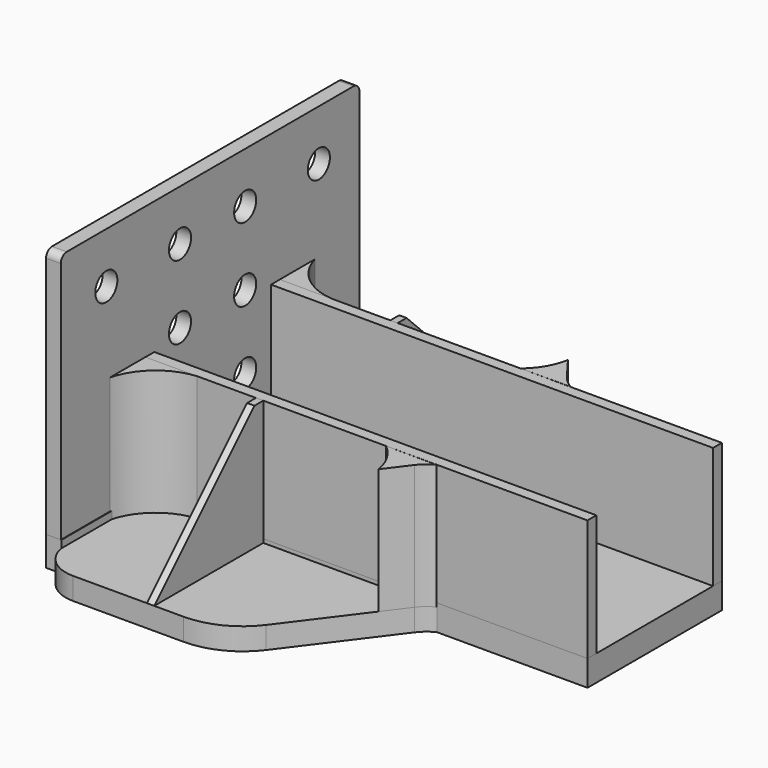
from build123d import *

# Parameters (mm, degrees)
F1_DEPTH   = 3.81
F2_W       = 2.54
F2_H       = 64.319235925
F3_DEPTH   = 44.45
F4_R       = 1.27
F5_R       = 1.27
F6_W       = 76.1874727905
F6_H       = 1.905
F7_DEPTH   = 25.4
F9_DEPTH   = 21.59
F11_DEPTH  = 21.59
F12_W      = 1.27
F12_H      = 23.495
F13_DEPTH  = 21.59
F14_SIZE   = 21.58999
F14_2_SIZE = 21.58999
F15_R      = 2.38125
F16_DEPTH  = 2.541
F17_W      = 78.74
F17_H      = 28.956
F18_DEPTH  = 4.445
F19_W      = 2.63135281
F19_H      = 18.218235925
F20_DEPTH  = 5.08


# Not quite as in the source:
# - a fillet or chamfer is up to 0.001 mm smaller than in the source, because OpenCascade refuses the exact size


with BuildPart() as f1:
    # F0 (on Top) → F1 (new body)
    with BuildSketch(Plane.XY):
        with BuildLine():
            Line((-38.1, 31.623), (-38.1, 12.573))
            Line((-38.1, 12.573), (12.7, 12.573))
            Line((12.7, 12.573), (38.1, 12.573))
            Line((38.1, 12.573), (38.1, 13.843))
            Line((38.1, 13.843), (14.9225, 13.843))
            ThreePointArc((14.9225, 13.843), (12.0826936686, 14.5133873372), (9.8425, 16.383))
            Line((9.8425, 16.383), (-2.54, 32.893))
            ThreePointArc((-2.54, 32.893), (-7.0203873372, 36.6322253257), (-12.7, 37.973))
            Line((-12.7, 37.973), (-31.75, 37.973))
            ThreePointArc((-31.75, 37.973), (-36.2401280605, 36.1131280605), (-38.1, 31.623))
        make_face()
    extrude(amount=F1_DEPTH)


with BuildPart() as f1b:
    # F0 (on Top) → F1, piece 2 (new body)
    with BuildSketch(Plane.XY):
        with BuildLine():
            Line((14.9225, -13.843), (38.1, -13.843))
            Line((38.1, -13.843), (38.1, -12.573))
            Line((38.1, -12.573), (12.7, -12.573))
            Line((12.7, -12.573), (-38.1, -12.573))
            Line((-38.1, -12.573), (-38.1, -31.623))
            ThreePointArc((-38.1, -31.623), (-36.2401280605, -36.1131280605), (-31.75, -37.973))
            Line((-31.75, -37.973), (-12.7, -37.973))
            ThreePointArc((-12.7, -37.973), (-7.0203873372, -36.6322253257), (-2.54, -32.893))
            Line((-2.54, -32.893), (9.8425, -16.383))
            ThreePointArc((9.8425, -16.383), (12.0826936686, -14.5133873372), (14.9225, -13.843))
        make_face()
    extrude(amount=F1_DEPTH)


with BuildPart() as f3:
    # F2 (on face) → F3 (new body)
    with BuildSketch(Plane.XY.offset(3.81)):
        with Locations((-39.37, -0.5366179625)):
            Rectangle(F2_W, F2_H)
    extrude(amount=F3_DEPTH)

    # F4
    f4_edges = [f3.edges().sort_by_distance(p)[0] for p in [
        (-39.37, 31.623, 48.26),
    ]]
    fillet(f4_edges, radius=F4_R)

    # F5
    f5_edges = [f3.edges().sort_by_distance(p)[0] for p in [
        (-39.37, -32.696236, 48.26),
    ]]
    fillet(f5_edges, radius=F5_R)

    # F15 (on face) → F16 (cut, through all)
    with BuildSketch(Plane.YZ.offset(-38.1)):
        with Locations((22.89175, 39.52875)):
            Circle(F15_R)
        with Locations((7.01675, 39.52875)):
            Circle(F15_R)
        with Locations((7.01675, 26.82875)):
            Circle(F15_R)
        with Locations((7.01675, 14.12875)):
            Circle(F15_R)
        with Locations((-22.89175, 39.52875)):
            Circle(F15_R)
        with Locations((-7.01675, 26.82875)):
            Circle(F15_R)
        with Locations((-7.01675, 14.12875)):
            Circle(F15_R)
        with Locations((-7.01675, 39.52875)):
            Circle(F15_R)
    extrude(amount=-F16_DEPTH, mode=Mode.SUBTRACT)


with BuildPart() as f7:
    # F6 (on Top) → F7 (new body)
    with BuildSketch(Plane.XY):
        with Locations((0.0062636048, 13.5255)):
            Rectangle(F6_W, F6_H)
    extrude(amount=F7_DEPTH)


with BuildPart() as f7b:
    # F6 (on Top) → F7, piece 2 (new body)
    with BuildSketch(Plane.XY):
        with Locations((0.0062636048, -13.5255)):
            Rectangle(F6_W, F6_H)
    extrude(amount=F7_DEPTH)


with BuildPart() as f9:
    # F8 (on face) → F9 (new body)
    with BuildSketch(Plane.XY.offset(3.81)):
        with BuildLine():
            ThreePointArc((-29.2110200971, 14.478), (-34.8634746859, 16.8788696345), (-38.1, 22.098))
            Line((-38.1, 22.098), (-38.1, 14.4734261557))
            Line((-38.1, 14.4734261557), (-29.2110200971, 14.478))
        make_face()
    extrude(amount=F9_DEPTH)


with BuildPart() as f9b:
    # F8 (on face) → F9, piece 2 (new body)
    with BuildSketch(Plane.XY.offset(3.81)):
        with BuildLine():
            Line((-38.1, -14.4734261557), (-38.1, -22.098))
            ThreePointArc((-38.1, -22.098), (-34.8634746859, -16.8788696345), (-29.2110200971, -14.478))
            Line((-29.2110200971, -14.478), (-38.1, -14.4734261557))
        make_face()
    extrude(amount=F9_DEPTH)


with BuildPart() as f11:
    # F10 (on face) → F11 (new body)
    with BuildSketch(Plane.XY.offset(3.81)):
        with BuildLine():
            ThreePointArc((6.8367980262, 20.3906026317), (5.6419248641, 17.1304778187), (3.4012782853, 14.478))
            Line((3.4012782853, 14.478), (12.0826936686, 14.5133873372))
            ThreePointArc((12.0826936686, 14.5133873372), (10.8537537608, 15.3177765137), (9.8425, 16.383))
            Line((9.8425, 16.383), (6.8367980262, 20.3906026317))
        make_face()
    extrude(amount=F11_DEPTH)


with BuildPart() as f11b:
    # F10 (on face) → F11, piece 2 (new body)
    with BuildSketch(Plane.XY.offset(3.81)):
        with BuildLine():
            Line((12.0826936686, -14.5133873372), (3.4012782853, -14.478))
            ThreePointArc((3.4012782853, -14.478), (5.6419248641, -17.1304778187), (6.8367980262, -20.3906026317))
            Line((6.8367980262, -20.3906026317), (9.8425, -16.383))
            ThreePointArc((9.8425, -16.383), (10.8537537608, -15.3177765137), (12.0826936686, -14.5133873372))
        make_face()
    extrude(amount=F11_DEPTH)


with BuildPart() as f13:
    # F12 (on face) → F13 (new body)
    with BuildSketch(Plane.XY.offset(3.81)):
        with Locations((-18.415, 26.2255)):
            Rectangle(F12_W, F12_H)
    extrude(amount=F13_DEPTH)

    # F14 (size 21.59 in the source; OpenCascade refuses exactly that, so slightly less here)
    f14_edges = [f13.edges().sort_by_distance(p)[0] for p in [
        (-18.415, 37.973, 25.4),
    ]]
    chamfer(f14_edges, length=F14_SIZE)


with BuildPart() as f13b:
    # F12 (on face) → F13, piece 2 (new body)
    with BuildSketch(Plane.XY.offset(3.81)):
        with Locations((-18.415, -26.2255)):
            Rectangle(F12_W, F12_H)
    extrude(amount=F13_DEPTH)

    # F14#2 (size 21.59 in the source; OpenCascade refuses exactly that, so slightly less here)
    f14_2_edges = [f13b.edges().sort_by_distance(p)[0] for p in [
        (-18.415, -37.973, 25.4),
    ]]
    chamfer(f14_2_edges, length=F14_2_SIZE)


with BuildPart() as f18:
    # F17 (on face) → F18 (new body)
    with BuildSketch(Plane(origin=(0, 0, 0), x_dir=(1, 0, 0), z_dir=(0, 0, -1))):
        with Locations((-1.27, 0)):
            Rectangle(F17_W, F17_H)
    extrude(amount=-F18_DEPTH)


with BuildPart() as f20:
    # F19 (on face) → F20 (new body)
    with BuildSketch(Plane(origin=(0, 0, 0), x_dir=(1, 0, 0), z_dir=(0, 0, -1))):
        with Locations((-39.324323595, 23.5871179625)):
            Rectangle(F19_W, F19_H)
    extrude(amount=-F20_DEPTH)


with BuildPart() as f20b:
    # F19 (on face) → F20, piece 2 (new body)
    with BuildSketch(Plane(origin=(0, 0, 0), x_dir=(1, 0, 0), z_dir=(0, 0, -1))):
        with Locations((-39.324323595, -23.5871179625)):
            Rectangle(F19_W, F19_H)
    extrude(amount=-F20_DEPTH)


solid = Compound([f1.part, f1b.part, f3.part, f7.part, f7b.part, f9.part, f9b.part, f11.part, f11b.part, f13.part, f13b.part, f18.part, f20.part, f20b.part])
